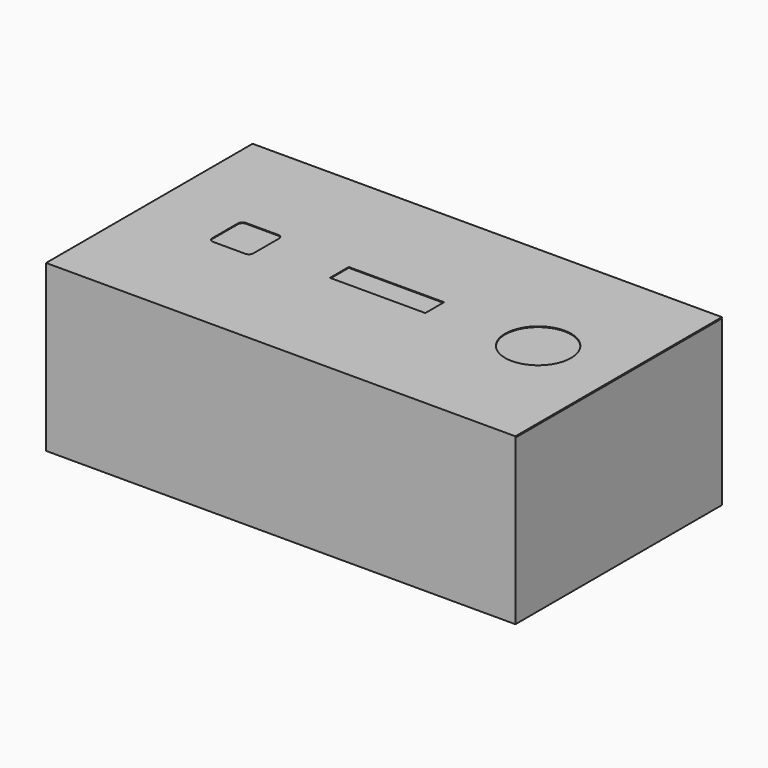
from build123d import *

# Parameters (mm, degrees)
F1_DEPTH = 127
F2_W     = 51.5939278
F2_H     = 12.7
F3_DEPTH = 0.4064


# Not quite as in the source:
# - the dataset's text gives a spline's control points without its knots; the knots are read off the source's solid


with BuildPart() as f1:
    # F0 (on Right) → F1 (new body, symmetric)
    with BuildSketch(Plane.YZ):
        Polygon((-139.7, 0), (0, 0), (0, 88.9), (-139.2936, 88.9), (-139.2936, 89.154), (0, 89.154), (0, 89.5604), (-139.7, 89.5604), align=None)
    extrude(amount=F1_DEPTH, both=True)

    # F2 (on face) → F3 (cut, through all)
    with BuildSketch(Plane.XY.offset(89.5604)):
        with BuildLine():
            add(Edge.make_bspline(
                [(-64.7785070788, -79.8723427679), (-64.3378678788, -79.4313733679), (-64.0812262788, -78.8116133679), (-64.0812262788, -78.1883989679)],
                knots=[1, 1, 1, 1, 2, 2, 2, 2], degree=3))
            Line((-64.0812262788, -78.1883989679), (-64.0812262788, -60.7258989679))
            add(Edge.make_bspline(
                [(-64.0812262788, -60.7258989679), (-64.0812262788, -60.1023289679), (-64.3378678788, -59.4828991679), (-64.7785070788, -59.0419297679)],
                knots=[0, 0, 0, 0, 1, 1, 1, 1], degree=3))
            add(Edge.make_bspline(
                [(-64.7785070788, -59.0419297679), (-65.2194764788, -58.6012905679), (-65.8385506788, -58.3446489679), (-66.4624762788, -58.3446489679)],
                knots=[1, 1, 1, 1, 2, 2, 2, 2], degree=3))
            Line((-66.4624762788, -58.3446489679), (-83.9249762788, -58.3446489679))
            add(Edge.make_bspline(
                [(-83.9249762788, -58.3446489679), (-84.5481906788, -58.3446489679), (-85.1675950788, -58.6012905679), (-85.6082342788, -59.0419297679), (-86.0492036788, -59.4828991679), (-86.3062262788, -60.1023289679), (-86.3062262788, -60.7258989679)],
                knots=[0, 0, 0, 0, 1, 1, 1, 2, 2, 2, 2], degree=3))
            Line((-86.3062262788, -60.7258989679), (-86.3062262788, -78.1883989679))
            add(Edge.make_bspline(
                [(-86.3062262788, -78.1883989679), (-86.3062262788, -78.8116133679), (-86.0492036788, -79.4313733679), (-85.6082342788, -79.8723427679)],
                knots=[0, 0, 0, 0, 1, 1, 1, 1], degree=3))
            add(Edge.make_bspline(
                [(-85.6082342788, -79.8723427679), (-85.1675950788, -80.3126517679), (-84.5481906788, -80.5696489679), (-83.9249762788, -80.5696489679)],
                knots=[1, 1, 1, 1, 2, 2, 2, 2], degree=3))
            Line((-83.9249762788, -80.5696489679), (-66.4624762788, -80.5696489679))
            add(Edge.make_bspline(
                [(-66.4624762788, -80.5696489679), (-65.8385506788, -80.5696489679), (-65.2194764788, -80.3126517679), (-64.7785070788, -79.8723427679)],
                knots=[0, 0, 0, 0, 1, 1, 1, 1], degree=3))
        make_face()
        with Locations((1.0063626212, -69.0602739679)):
            Rectangle(F2_W, F2_H)
        with BuildLine():
            add(Edge.make_bspline(
                [(95.3862221212, -56.4057399679), (92.0802851212, -53.0994727679), (87.4335837212, -51.1747369679), (82.7579009212, -51.1747369679)],
                knots=[7, 7, 7, 7, 8, 8, 8, 8], degree=3))
            add(Edge.make_bspline(
                [(82.7579009212, -51.1747369679), (78.0822181212, -51.1747369679), (73.4354659212, -53.0994727679), (70.1295543212, -56.4057399679)],
                knots=[0, 0, 0, 0, 1, 1, 1, 1], degree=3))
            add(Edge.make_bspline(
                [(70.1295543212, -56.4057399679), (66.8236173212, -59.7116769679), (64.8985259212, -64.3587339679), (64.8985259212, -69.0341119679), (64.8985259212, -73.7097947679), (66.8236173212, -78.3564961679), (70.1295543212, -81.6631189679)],
                knots=[1, 1, 1, 1, 2, 2, 2, 3, 3, 3, 3], degree=3))
            add(Edge.make_bspline(
                [(70.1295543212, -81.6631189679), (73.4354659212, -84.9690305679), (78.0822181212, -86.8934869679), (82.7579009212, -86.8934869679), (87.4335837212, -86.8934869679), (92.0802851212, -84.9690305679), (95.3862221212, -81.6631189679)],
                knots=[3, 3, 3, 3, 4, 4, 4, 5, 5, 5, 5], degree=3))
            add(Edge.make_bspline(
                [(95.3862221212, -81.6631189679), (98.6928195212, -78.3564961679), (100.6172759212, -73.7097947679), (100.6172759212, -69.0341119679), (100.6172759212, -64.3587339679), (98.6928195212, -59.7116769679), (95.3862221212, -56.4057399679)],
                knots=[5, 5, 5, 5, 6, 6, 6, 7, 7, 7, 7], degree=3))
        make_face()
    extrude(amount=-F3_DEPTH, mode=Mode.SUBTRACT)


solid = f1.part
